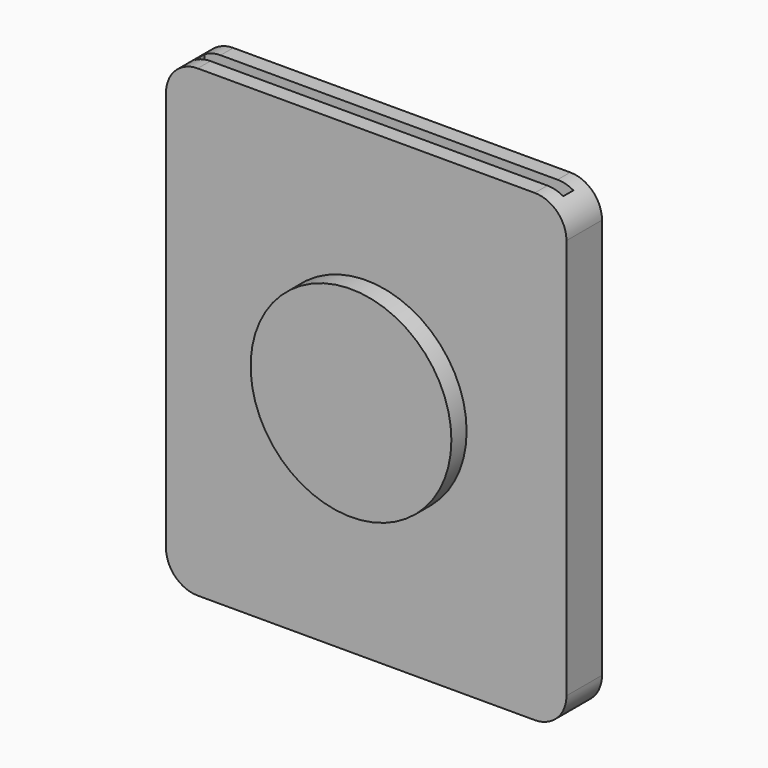
from build123d import *

# Parameters (mm, degrees)
F0_W        = 63.1147548556
F0_H        = 73.1557384133
F1_DEPTH    = 7
F2_R        = 15.8223055834
F3_DEPTH    = 3
F4_T        = -2.5
F5_T1_DEPTH = 32


# Not quite as in the source:
# - a fillet or chamfer that OpenCascade refuses, or shapes differently, is made with other operations: its cross-section is extruded or revolved along the edge and cut away or added


with BuildPart() as f1:
    # F0 (on Front) → F1 (new body)
    with BuildSketch(Plane.XZ):
        Rectangle(F0_W, F0_H)
    extrude(amount=F1_DEPTH)

    # F2 (on face) → F3 (join)
    with BuildSketch(Plane.XZ.offset(7)):
        Circle(F2_R)
    extrude(amount=F3_DEPTH)

    # F4
    f4_openings = [f1.faces().sort_by_distance(p)[0] for p in [
        (0, -3.5, 36.577869),
    ]]
    offset(amount=F4_T, openings=f4_openings, kind=Kind.INTERSECTION)

    # F5: fillet of radius 5 on 4 edges, made by hand

    # F5_s2 → F5_t1 (cut)
    with BuildSketch(Plane.XZ.offset(-12.5)):
        with BuildLine():
            ThreePointArc((31.5573774278, 31.5778692067), (30.0929113337, 35.1134031126), (26.5573774278, 36.5778692067))
            Line((26.5573774278, 36.5778692067), (31.5573774278, 36.5778692067))
            Line((31.5573774278, 36.5778692067), (31.5573774278, 31.5778692067))
        make_face()
        with BuildLine():
            ThreePointArc((31.5573774278, -31.5778692067), (30.0929113337, -35.1134031126), (26.5573774278, -36.5778692067))
            Line((26.5573774278, -36.5778692067), (31.5573774278, -36.5778692067))
            Line((31.5573774278, -36.5778692067), (31.5573774278, -31.5778692067))
        make_face()
        with BuildLine():
            ThreePointArc((-31.5573774278, -31.5778692067), (-30.0929113337, -35.1134031126), (-26.5573774278, -36.5778692067))
            Line((-26.5573774278, -36.5778692067), (-31.5573774278, -36.5778692067))
            Line((-31.5573774278, -36.5778692067), (-31.5573774278, -31.5778692067))
        make_face()
        with BuildLine():
            ThreePointArc((-31.5573774278, 31.5778692067), (-30.0929113337, 35.1134031126), (-26.5573774278, 36.5778692067))
            Line((-26.5573774278, 36.5778692067), (-31.5573774278, 36.5778692067))
            Line((-31.5573774278, 36.5778692067), (-31.5573774278, 31.5778692067))
        make_face()
    extrude(amount=F5_T1_DEPTH, mode=Mode.SUBTRACT)


solid = f1.part
